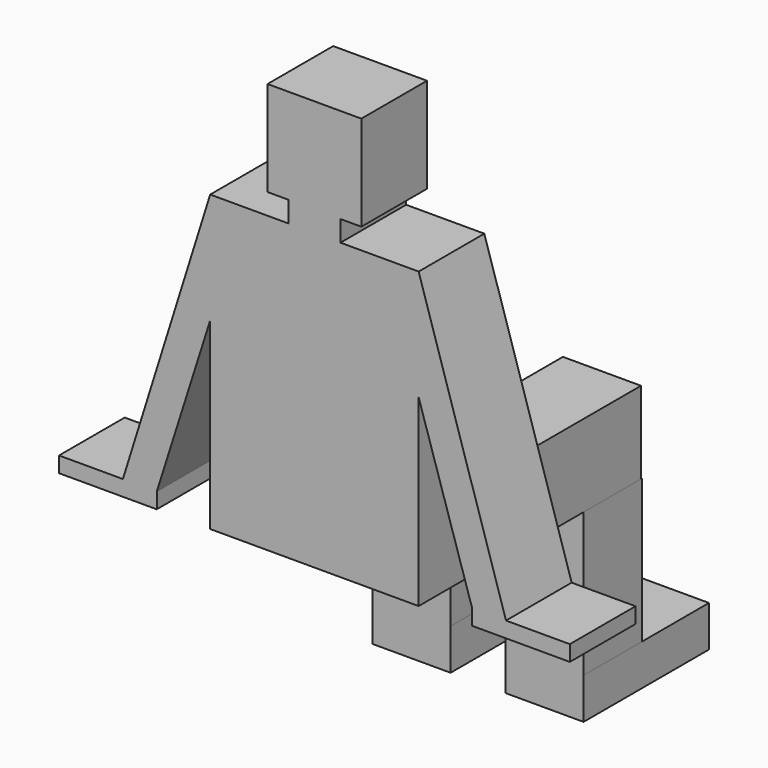
from build123d import *

# Parameters (mm, degrees)
F1_DEPTH = 20
F2_W     = 19.0279083326
F2_H     = 47.3126359284
F3_DEPTH = 20
F4_W     = 19.0279083326
F4_H     = 17.7422408015
F5_DEPTH = 35
F6_W     = 19.0279087983
F6_H     = 38.1843838841
F6_H_2   = 17.7422408015
F7_DEPTH = 10


# Not quite as in the source:
# - ends of sketch curves that miss each other by under 0.0002 mm in the source are joined


with BuildPart() as f1:
    # F0 (on Front) → F1 (new body)
    with BuildSketch(Plane.XZ):
        Polygon((-6.3491990761, 71.7460297603), (-25.3968193009, 71.7460297603), (-46.6666553218, 3.8095274944), (-62.2222101619, 3.8095274944), (-62.2222101619, 0), (-38.4126887615, 0), (-38.4126887615, 3.8095274944), (-25.3968193009, 44.7619079595), (-25.3968193009, 0), (0, 0), (25.3968193009, 0), (25.3968193009, 44.7619079595), (38.4126887615, 3.8095274944), (38.4126887615, 0), (62.2222101619, 0), (62.2222101619, 3.8095274944), (46.6666553218, 3.8095274944), (25.3968193009, 71.7460297603), (6.3491990761, 71.7460297603), (6.3491990761, 76.8254005194), (11.4285635112, 76.8254005194), (11.4285635112, 100), (0, 100), (-11.4285635112, 100), (-11.4285635112, 76.8254005194), (-6.3491990761, 76.8254005194), align=None)
    extrude(amount=F1_DEPTH)

    # F2 (on Top) → F3 (join)
    with BuildSketch(Plane.XY):
        with Locations((-16.1994355731, 23.6563179642)):
            Rectangle(F2_W, F2_H)
        with Locations((16.1994355731, 23.6563179642)):
            Rectangle(F2_W, F2_H)
    extrude(amount=F3_DEPTH)

    # F4 (on Top) → F5 (join)
    with BuildSketch(Plane.XY):
        with Locations((16.1994318478, 38.6986536905)):
            Rectangle(F4_W, F4_H)
        with Locations((-16.1994318478, 38.6986536905)):
            Rectangle(F4_W, F4_H)
    extrude(amount=-F5_DEPTH)

    # F6 (on face) → F7 (join)
    with BuildSketch(Plane(origin=(0, 0, -35), x_dir=(1, 0, 0), z_dir=(0, 0, -1))):
        Polygon((25.7133860141, -68.0119171739), (25.7133860141, -47.5697740912), (6.6854776815, -47.5697740912), (6.6854772158, -68.0119171739), align=None)
        with Locations((-16.199431615, -48.9197252318)):
            Rectangle(F6_W, F6_H)
        with Locations((16.199431615, -38.6986536905)):
            Rectangle(F6_W, F6_H_2)
    extrude(amount=F7_DEPTH)


solid = f1.part
